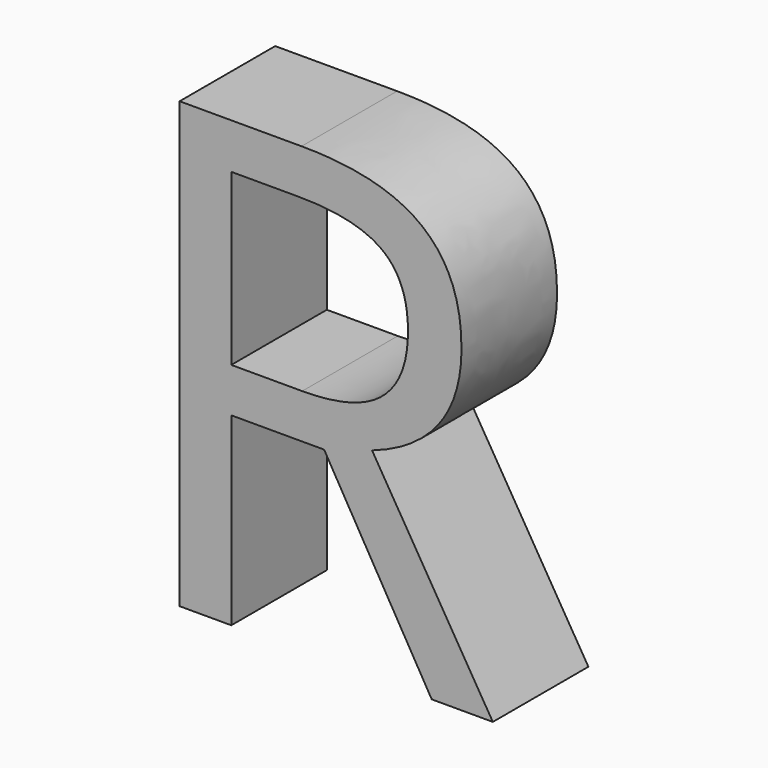
from build123d import *

# Parameters (mm, degrees)
F0_TEXT_SIZE = 132.4309191356
F1_DEPTH     = 25.4


# Not quite as in the source:
# - Text() gives the source's letters only with a copy of the font that has no kerning and outlines rounded to 1/6400 em; it was checked with that copy


with BuildPart() as f1:
    # F0 (on Front) → F1 (new body)
    with BuildSketch(Plane.XZ):
        with Locations((-53.6909215152, -50.9838163853)):
            Text('R', F0_TEXT_SIZE, font='Open Sans', text_align=(TextAlign.LEFT, TextAlign.BOTTOM))
    extrude(amount=F1_DEPTH)


solid = f1.part
